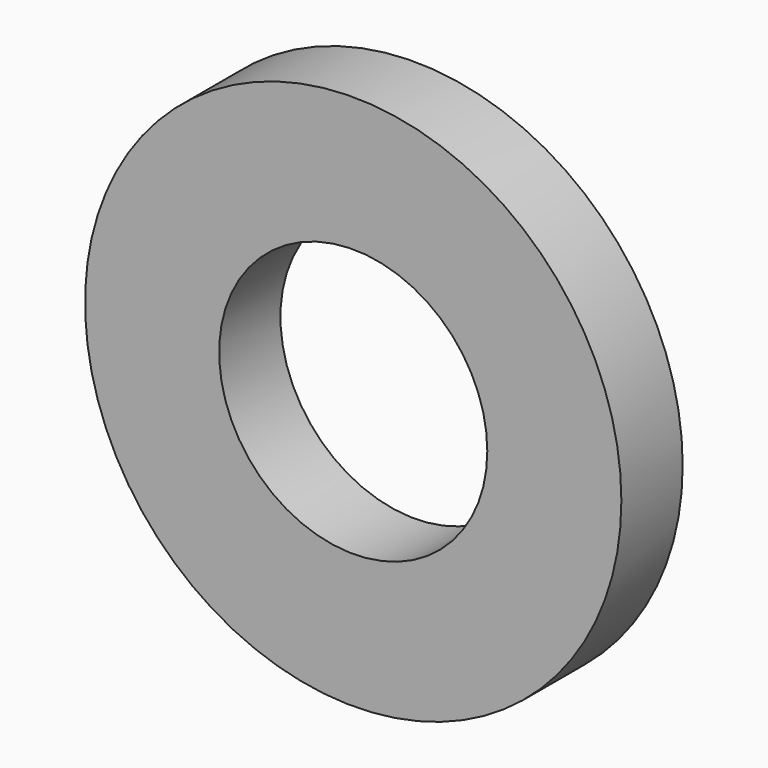
from build123d import *

# Parameters (mm, degrees)
F0_R     = 35
F0_R_2   = 17.5
F2_DEPTH = 10


# Not quite as in the source:
# - the program builds the solid bodies; features that only make, move or delete a surface that nothing else refers to are left out


with BuildPart() as f2:
    # F0 (on Front) → F2 (new body)
    with BuildSketch(Plane.XZ):
        Circle(F0_R)
        Circle(F0_R_2, mode=Mode.SUBTRACT)
    extrude(amount=F2_DEPTH)


solid = f2.part
